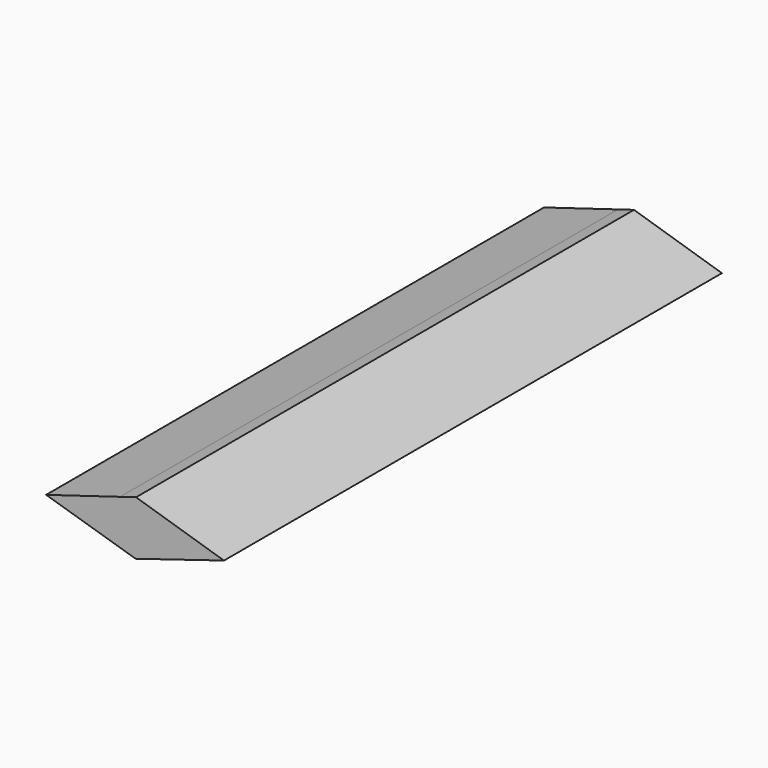
from build123d import *

# Parameters (mm, degrees)
F1_DEPTH = 25.4
F2_DEPTH = 508


with BuildPart() as f1:
    # F0 (on Front) → F1 (new body)
    with BuildSketch(Plane.XZ):
        with BuildLine():
            Line((-23.26887446, 0), (23.26887446, 0))
            ThreePointArc((23.26887446, 0), (20.4736338233, 11.0576144219), (12.7594845956, 19.4585732131))
            Line((12.7594845956, 19.4585732131), (0.4321157806, 23.2648618003))
            Line((0.4321157806, 23.2648618003), (-13.2265486778, 19.1441617396))
            ThreePointArc((-13.2265486778, 19.1441617396), (-20.6059144344, 10.8091076855), (-23.26887446, 0))
        make_face()
        with BuildLine():
            Line((75.7796689868, 0), (23.26887446, 0))
            ThreePointArc((23.26887446, 0), (20.5584527971, -10.8991071756), (13.0586223544, -19.2590991701))
            Line((13.0586223544, -19.2590991701), (75.7796689868, 0))
        make_face()
        with BuildLine():
            ThreePointArc((12.7594845956, 19.4585732131), (20.4736338233, 11.0576144219), (23.26887446, 0))
            Line((23.26887446, 0), (75.7796689868, 0))
            Line((75.7796689868, 0), (12.7594845956, 19.4585732131))
        make_face()
        with BuildLine():
            ThreePointArc((13.0586223544, -19.2590991701), (20.5584527971, -10.8991071756), (23.26887446, 0))
            Line((23.26887446, 0), (-23.26887446, 0))
            ThreePointArc((-23.26887446, 0), (-20.5222893701, -10.9670487209), (-12.9309307101, -19.3450652521))
            Line((-12.9309307101, -19.3450652521), (0, -23.26887446))
            Line((0, -23.26887446), (13.0586223544, -19.2590991701))
        make_face()
        with BuildLine():
            Line((-76.6826793551, 0), (-23.26887446, 0))
            ThreePointArc((-23.26887446, 0), (-20.6059144344, 10.8091076855), (-13.2265486778, 19.1441617396))
            Line((-13.2265486778, 19.1441617396), (-76.6826793551, 0))
        make_face()
        with BuildLine():
            ThreePointArc((-12.9309307101, -19.3450652521), (-20.5222893701, -10.9670487209), (-23.26887446, 0))
            Line((-23.26887446, 0), (-76.6826793551, 0))
            Line((-76.6826793551, 0), (-12.9309307101, -19.3450652521))
        make_face()
    extrude(amount=F1_DEPTH)

    # F2 (add): a face of the model
    f2_faces = [f1.faces().sort_by_distance(p)[0] for p in [
        (-0.2289903697, -25.4, -0.0013375532),
    ]]
    extrude(f2_faces, amount=F2_DEPTH)


solid = f1.part
